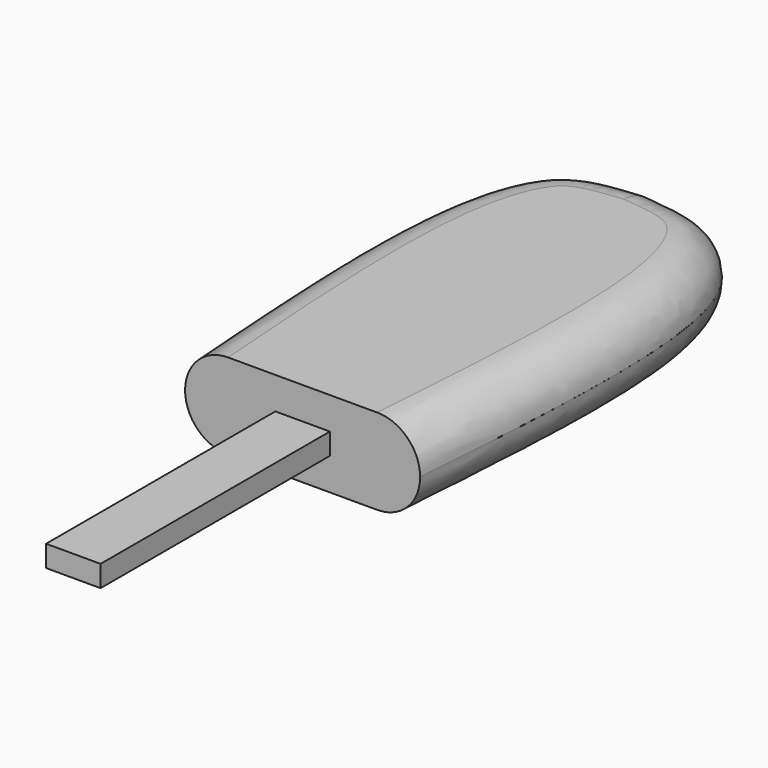
from build123d import *

# Parameters (mm, degrees)
F1_DEPTH = 5
F2_R     = 4.999
F4_DEPTH = 1.25


# Not quite as in the source:
# - a fillet or chamfer is up to 0.001 mm smaller than in the source, because OpenCascade refuses the exact size


with BuildPart() as f1:
    # F0 (on Top) → F1 (new body, symmetric)
    with BuildSketch(Plane.XY):
        with BuildLine():
            add(Edge.make_bspline(
                [(-13.7097453699, 0), (-14.7537661126, 14.3834786699), (-16.3965507437, 37.0161302377), (-10.0715641044, 50.9942741703), (-3.1640643241, 51.6181998618), (0, 51.9039966166)],
                knots=[0, 0, 0, 0, 0.4858446106, 0.7644848677, 1, 1, 1, 1], degree=3))
            Line((-13.7097453699, 0), (13.7097453699, 0))
            add(Edge.make_bspline(
                [(13.7097453699, 0), (14.7537661126, 14.3834786699), (16.3965507437, 37.0161302377), (10.0715641044, 50.9942741703), (3.1640643241, 51.6181998618), (0, 51.9039966166)],
                knots=[0, 0, 0, 0, 0.4858446106, 0.7644848677, 1, 1, 1, 1], degree=3))
        make_face()
    extrude(amount=F1_DEPTH, both=True)

    # F2 (radius 5 in the source; OpenCascade refuses exactly that, so slightly less here)
    f2_edges = [f1.edges().sort_by_distance(p)[0] for p in [
        (-14.960078, 30.185645, 5),
        (14.960078, 30.185645, 5),
        (-14.960078, 30.185645, -5),
        (14.960078, 30.185645, -5),
    ]]
    fillet(f2_edges, radius=F2_R)

    # F3 (on Top) → F4 (join, symmetric)
    with BuildSketch(Plane.XY):
        Polygon((3.1797995325, 15.8989857882), (0, 15.8989857882), (-3.1797995325, 15.8989857882), (-3.1797995325, -33.4308445454), (0, -33.4308445454), (3.1797995325, -33.4308445454), align=None)
    extrude(amount=F4_DEPTH, both=True)


solid = f1.part
